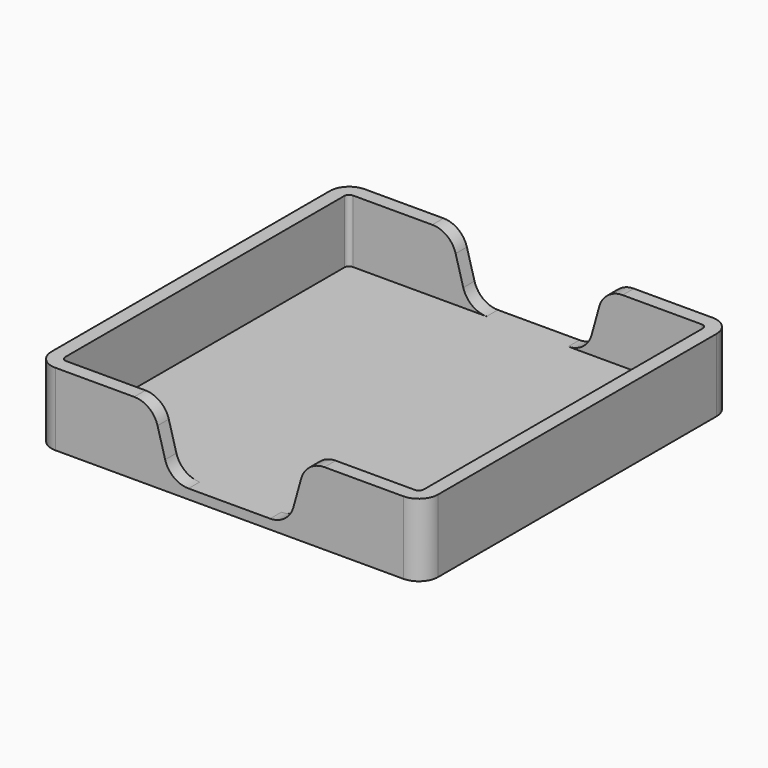
from build123d import *

# Parameters (mm, degrees)
F0_W      = 79.8
F0_H      = 79.8
F1_DEPTH  = 15
F2_W      = 74
F2_H      = 74
F3_DEPTH  = 13
F4_W      = 73.8
F4_H      = 73.8
F4_W_2    = 69.8
F4_H_2    = 69.8
F5_DEPTH  = 2
F7_DEPTH  = 2
F8_R      = 2
F9_R      = 4
F10_R     = 0.99999
F12_DEPTH = 79.801
F13_R     = 5
F14_R     = 4
F15_R     = 1


# Not quite as in the source:
# - a fillet or chamfer is up to 0.001 mm smaller than in the source, because OpenCascade refuses the exact size


with BuildPart() as f1:
    # F0 (on Top) → F1 (new body)
    with BuildSketch(Plane.XY):
        Rectangle(F0_W, F0_H)
    extrude(amount=F1_DEPTH)

    # F2 (on face) → F3 (cut)
    with BuildSketch(Plane.XY.offset(15)):
        Rectangle(F2_W, F2_H)
    extrude(amount=-F3_DEPTH, mode=Mode.SUBTRACT)

    # F4 (on face) → F5 (join)
    with BuildSketch(Plane(origin=(0, 0, 0), x_dir=(1, 0, 0), z_dir=(0, 0, -1))):
        Rectangle(F4_W, F4_H)
        Rectangle(F4_W_2, F4_H_2, mode=Mode.SUBTRACT)
    extrude(amount=F5_DEPTH)

    # F6 (on face) → F7 (cut, through all)
    with BuildSketch(Plane(origin=(0, 0, -2), x_dir=(1, 0, 0), z_dir=(0, 0, -1))):
        Polygon((36.9, -21.9), (36.9, 21.9), (21.9, 21.9), (21.9, 36.9), (-21.9, 36.9), (-21.9, 21.9), (-36.9, 21.9), (-36.9, -21.9), (-21.9, -21.9), (-21.9, -36.9), (21.9, -36.9), (21.9, -21.9), align=None)
    extrude(amount=-F7_DEPTH, mode=Mode.SUBTRACT)

    # F8
    f8_edges = [f1.edges().sort_by_distance(p)[0] for p in [
        (-34.9, 34.9, -1),
        (-34.9, -34.9, -1),
        (34.9, -34.9, -1),
        (34.9, 34.9, -1),
    ]]
    fillet(f8_edges, radius=F8_R)

    # F9
    f9_edges = [f1.edges().sort_by_distance(p)[0] for p in [
        (-36.9, 36.9, -1),
        (36.9, 36.9, -1),
        (36.9, -36.9, -1),
        (-36.9, -36.9, -1),
    ]]
    fillet(f9_edges, radius=F9_R)

    # F10 (radius 1 in the source; OpenCascade refuses exactly that, so slightly less here)
    f10_edges = [f1.edges().sort_by_distance(p)[0] for p in [
        (21.9, -35.9, -2),
        (21.9, -35.9, 0),
        (35.9, -21.9, -2),
        (35.9, -21.9, 0),
        (-35.9, -21.9, -2),
        (-35.9, -21.9, 0),
        (-21.9, -35.9, -2),
        (-21.9, -35.9, 0),
        (-35.9, 21.9, -2),
        (-35.9, 21.9, 0),
        (-21.9, 35.9, -2),
        (-21.9, 35.9, 0),
        (21.9, 35.9, -2),
        (21.9, 35.9, 0),
        (35.9, 21.9, -2),
        (35.9, 21.9, 0),
    ]]
    fillet(f10_edges, radius=F10_R)

    # F11 (on face) → F12 (cut, through all)
    with BuildSketch(Plane.XZ.offset(39.9)):
        Polygon((20, 30), (-20, 30), (-12.2222222222, 2), (12.2222222222, 2), align=None)
    extrude(amount=-F12_DEPTH, mode=Mode.SUBTRACT)

    # F13
    f13_edges = [f1.edges().sort_by_distance(p)[0] for p in [
        (-15.833333, 38.45, 15),
        (-15.833333, -38.45, 15),
        (15.833333, -38.45, 15),
        (15.833333, 38.45, 15),
        (-12.222222, 38.45, 2),
        (-12.222222, -38.45, 2),
        (12.222222, -38.45, 2),
        (12.222222, 38.45, 2),
    ]]
    fillet(f13_edges, radius=F13_R)

    # F14
    f14_edges = [f1.edges().sort_by_distance(p)[0] for p in [
        (39.9, -39.9, 7.5),
        (39.9, 39.9, 7.5),
        (-39.9, -39.9, 7.5),
        (-39.9, 39.9, 7.5),
    ]]
    fillet(f14_edges, radius=F14_R)

    # F15
    f15_edges = [f1.edges().sort_by_distance(p)[0] for p in [
        (37, 37, 8.5),
        (-37, 37, 8.5),
        (-37, -37, 8.5),
        (37, -37, 8.5),
    ]]
    fillet(f15_edges, radius=F15_R)


solid = f1.part
